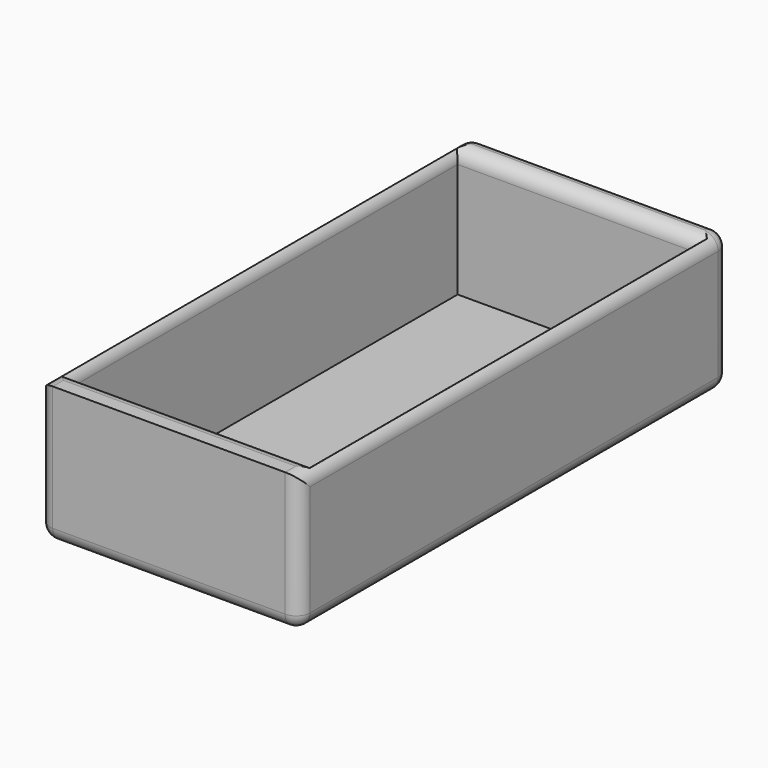
from build123d import *

# Parameters (mm, degrees)
F0_W          = 95.25
F0_H          = 196.85
F1_DEPTH      = 50.8
F2_W          = 87.2193016112
F2_H          = 177.3245334625
F3_DEPTH      = 46.99
F4_T1_DEPTH   = 204.47
F4_T3_DEPTH   = 85.09
F4_T5_DEPTH   = 40.64
F4_T7_DEPTH   = 186.69
F4_T9_DEPTH   = 58.42
F4_T11_DEPTH  = 87.2193016112
F4_T13_DEPTH  = 177.3245334625
F4_S17_W      = 5.1816
F4_S17_H      = 5.1816
F4_T18_DEPTH  = 5.1816
F4_S23_W      = 5.1816
F4_S23_H      = 5.1816
F4_T24_DEPTH  = 5.1816
F4_S29_W      = 5.1816
F4_S29_H      = 5.1816
F4_T30_DEPTH  = 5.1816
F4_S35_W      = 5.1816
F4_S35_H      = 5.1816
F4_T36_DEPTH  = 5.1816
F4_S41_W      = 5.1816
F4_S41_H      = 5.1816
F4_T42_DEPTH  = 5.1816
F4_S47_W      = 5.1816
F4_S47_H      = 5.1816
F4_T48_DEPTH  = 5.1816
F4_T55_DEPTH  = 99.9193016112
F4_T60_DEPTH  = 190.0245334625
F4_T69_DEPTH  = 99.9193016112
F4_T74_DEPTH  = 190.0245334625
F4_T83_DEPTH  = 190.0245334625
F4_T89_DEPTH  = 99.9193016112
F4_T97_DEPTH  = 99.9193016112
F4_T102_DEPTH = 190.0245334625


# Not quite as in the source:
# - a fillet or chamfer that OpenCascade refuses, or shapes differently, is made with other operations: its cross-section is extruded or revolved along the edge and cut away or added


with BuildPart() as f1:
    # F0 (on Top) → F1 (new body)
    with BuildSketch(Plane.XY):
        Rectangle(F0_W, F0_H)
    extrude(amount=F1_DEPTH)

    # F2 (on face) → F3 (cut)
    with BuildSketch(Plane.XY.offset(50.8)):
        with Locations((-0.4809889942, 0.1569911838)):
            Rectangle(F2_W, F2_H)
    extrude(amount=-F3_DEPTH, mode=Mode.SUBTRACT)

    # F4: fillet of radius 5.08 on 15 edges, made by hand

    # F4_s2 → F4_t1 (cut)
    with BuildSketch(Plane.XZ.offset(-93.345)):
        with BuildLine():
            ThreePointArc((-47.625, 45.72), (-46.1371024484, 49.3121024484), (-42.545, 50.8))
            Line((-42.545, 50.8), (-47.625, 50.8))
            Line((-47.625, 50.8), (-47.625, 45.72))
        make_face()
        with BuildLine():
            ThreePointArc((47.625, 45.72), (46.1371024484, 49.3121024484), (42.545, 50.8))
            Line((42.545, 50.8), (47.625, 50.8))
            Line((47.625, 50.8), (47.625, 45.72))
        make_face()
    extrude(amount=F4_T1_DEPTH, mode=Mode.SUBTRACT)

    # F4_s4 → F4_t3 (cut)
    with BuildSketch(Plane.YZ.offset(-42.545)):
        with BuildLine():
            ThreePointArc((98.425, 45.72), (96.9371024484, 49.3121024484), (93.345, 50.8))
            Line((93.345, 50.8), (98.425, 50.8))
            Line((98.425, 50.8), (98.425, 45.72))
        make_face()
        with BuildLine():
            ThreePointArc((-93.345, 0), (-96.9371024484, 1.4878975516), (-98.425, 5.08))
            Line((-98.425, 5.08), (-98.425, 0))
            Line((-98.425, 0), (-93.345, 0))
        make_face()
        with BuildLine():
            ThreePointArc((98.425, 5.08), (96.9371024484, 1.4878975516), (93.345, 0))
            Line((93.345, 0), (98.425, 0))
            Line((98.425, 0), (98.425, 5.08))
        make_face()
    extrude(amount=F4_T3_DEPTH, mode=Mode.SUBTRACT)

    # F4_s6 → F4_t5 (cut)
    with BuildSketch(Plane.XY.offset(5.08)):
        with BuildLine():
            ThreePointArc((-42.545, 98.425), (-46.1371024484, 96.9371024484), (-47.625, 93.345))
            Line((-47.625, 93.345), (-47.625, 98.425))
            Line((-47.625, 98.425), (-42.545, 98.425))
        make_face()
        with BuildLine():
            ThreePointArc((42.545, 98.425), (46.1371024484, 96.9371024484), (47.625, 93.345))
            Line((47.625, 93.345), (47.625, 98.425))
            Line((47.625, 98.425), (42.545, 98.425))
        make_face()
    extrude(amount=F4_T5_DEPTH, mode=Mode.SUBTRACT)

    # F4_s8 → F4_t7 (cut)
    with BuildSketch(Plane.XZ.offset(-93.345)):
        with BuildLine():
            ThreePointArc((-47.625, 5.08), (-46.1371024484, 1.4878975516), (-42.545, 0))
            Line((-42.545, 0), (-47.625, 0))
            Line((-47.625, 0), (-47.625, 5.08))
        make_face()
        with BuildLine():
            ThreePointArc((47.625, 5.08), (46.1371024484, 1.4878975516), (42.545, 0))
            Line((42.545, 0), (47.625, 0))
            Line((47.625, 0), (47.625, 5.08))
        make_face()
    extrude(amount=F4_T7_DEPTH, mode=Mode.SUBTRACT)

    # F4_s10 → F4_t9 (cut)
    with BuildSketch(Plane.XY.offset(5.08)):
        with BuildLine():
            ThreePointArc((-47.625, -93.345), (-46.1371024484, -96.9371024484), (-42.545, -98.425))
            Line((-42.545, -98.425), (-47.625, -98.425))
            Line((-47.625, -98.425), (-47.625, -93.345))
        make_face()
        with BuildLine():
            ThreePointArc((47.625, -93.345), (46.1371024484, -96.9371024484), (42.545, -98.425))
            Line((42.545, -98.425), (47.625, -98.425))
            Line((47.625, -98.425), (47.625, -93.345))
        make_face()
    extrude(amount=F4_T9_DEPTH, mode=Mode.SUBTRACT)

    # F4_s12 → F4_t11 (cut)
    with BuildSketch(Plane.YZ.offset(-44.0906397998)):
        with BuildLine():
            ThreePointArc((93.899257915, 50.8), (90.3071554666, 49.3121024484), (88.819257915, 45.72))
            Line((88.819257915, 45.72), (88.819257915, 50.8))
            Line((88.819257915, 50.8), (93.899257915, 50.8))
        make_face()
        with BuildLine():
            ThreePointArc((-93.5852755475, 50.8), (-89.9931730991, 49.3121024484), (-88.5052755475, 45.72))
            Line((-88.5052755475, 45.72), (-88.5052755475, 50.8))
            Line((-88.5052755475, 50.8), (-93.5852755475, 50.8))
        make_face()
    extrude(amount=F4_T11_DEPTH, mode=Mode.SUBTRACT)

    # F4_s14 → F4_t13 (cut)
    with BuildSketch(Plane.XZ.offset(-88.819257915)):
        with BuildLine():
            ThreePointArc((-49.1706397998, 50.8), (-45.5785373514, 49.3121024484), (-44.0906397998, 45.72))
            Line((-44.0906397998, 45.72), (-44.0906397998, 50.8))
            Line((-44.0906397998, 50.8), (-49.1706397998, 50.8))
        make_face()
        with BuildLine():
            ThreePointArc((48.2086618114, 50.8), (44.6165593629, 49.3121024484), (43.1286618114, 45.72))
            Line((43.1286618114, 45.72), (43.1286618114, 50.8))
            Line((43.1286618114, 50.8), (48.2086618114, 50.8))
        make_face()
    extrude(amount=F4_T13_DEPTH, mode=Mode.SUBTRACT)


with BuildPart() as f4_tool16:
    # F4_s17 → F4_t18 (new body)
    with BuildSketch(Plane.XZ.offset(-93.345)):
        with Locations((-45.1358, 48.3108)):
            Rectangle(F4_S17_W, F4_S17_H)
    extrude(amount=-F4_T18_DEPTH)

    # F4_s19 → F4_t20 (revolve, cut)
    with BuildSketch(Plane(origin=(-42.545, 93.345, 45.72), x_dir=(0.7071067812, 0, -0.7071067812), z_dir=(0.7071067812, 0, 0.7071067812))):
        with BuildLine():
            ThreePointArc((0, -5.08), (5.08, 0), (0, 5.08))
            Line((0, 5.08), (0, -5.08))
        make_face()
    revolve(axis=Axis((-42.545, 93.345, 45.72), (0, 1, 0)), mode=Mode.SUBTRACT)


with BuildPart() as f1_1:
    add(f1.part)

    # F4_t15: cut F4_tool16
    add(f4_tool16.part, mode=Mode.SUBTRACT)


with BuildPart() as f4_tool22:
    # F4_s23 → F4_t24 (new body)
    with BuildSketch(Plane.XZ.offset(-93.345)):
        with Locations((45.1358, 48.3108)):
            Rectangle(F4_S23_W, F4_S23_H)
    extrude(amount=-F4_T24_DEPTH)

    # F4_s25 → F4_t26 (revolve, cut)
    with BuildSketch(Plane(origin=(42.545, 93.345, 45.72), x_dir=(-0.7071067812, 0, -0.7071067812), z_dir=(0.7071067812, 0, -0.7071067812))):
        with BuildLine():
            ThreePointArc((0, -5.08), (5.08, 0), (0, 5.08))
            Line((0, 5.08), (0, -5.08))
        make_face()
    revolve(axis=Axis((42.545, 93.345, 45.72), (0, 1, 0)), mode=Mode.SUBTRACT)


with BuildPart() as f1_2:
    add(f1_1.part)

    # F4_t21: cut F4_tool22
    add(f4_tool22.part, mode=Mode.SUBTRACT)


with BuildPart() as f4_tool28:
    # F4_s29 → F4_t30 (new body)
    with BuildSketch(Plane.XZ.offset(-93.345)):
        with Locations((-45.1358, 2.4892)):
            Rectangle(F4_S29_W, F4_S29_H)
    extrude(amount=-F4_T30_DEPTH)

    # F4_s31 → F4_t32 (revolve, cut)
    with BuildSketch(Plane(origin=(-42.545, 93.345, 5.08), x_dir=(0.7071067812, 0, 0.7071067812), z_dir=(-0.7071067812, 0, 0.7071067812))):
        with BuildLine():
            ThreePointArc((0, -5.08), (5.08, 0), (0, 5.08))
            Line((0, 5.08), (0, -5.08))
        make_face()
    revolve(axis=Axis((-42.545, 93.345, 5.08), (0, 1, 0)), mode=Mode.SUBTRACT)


with BuildPart() as f1_3:
    add(f1_2.part)

    # F4_t27: cut F4_tool28
    add(f4_tool28.part, mode=Mode.SUBTRACT)


with BuildPart() as f4_tool34:
    # F4_s35 → F4_t36 (new body)
    with BuildSketch(Plane.YZ.offset(-42.545)):
        with Locations((-95.9358, 2.4892)):
            Rectangle(F4_S35_W, F4_S35_H)
    extrude(amount=-F4_T36_DEPTH)

    # F4_s37 → F4_t38 (revolve, cut)
    with BuildSketch(Plane(origin=(-42.545, -93.345, 5.08), x_dir=(0, 0.7071067812, 0.7071067812), z_dir=(0, -0.7071067812, 0.7071067812))):
        with BuildLine():
            ThreePointArc((0, -5.08), (5.08, 0), (0, 5.08))
            Line((0, 5.08), (0, -5.08))
        make_face()
    revolve(axis=Axis((-42.545, -93.345, 5.08), (-1, 0, 0)), mode=Mode.SUBTRACT)


with BuildPart() as f1_4:
    add(f1_3.part)

    # F4_t33: cut F4_tool34
    add(f4_tool34.part, mode=Mode.SUBTRACT)


with BuildPart() as f4_tool40:
    # F4_s41 → F4_t42 (new body)
    with BuildSketch(Plane.YZ.offset(42.545)):
        with Locations((-95.9358, 2.4892)):
            Rectangle(F4_S41_W, F4_S41_H)
    extrude(amount=F4_T42_DEPTH)

    # F4_s43 → F4_t44 (revolve, cut)
    with BuildSketch(Plane(origin=(42.545, -93.345, 5.08), x_dir=(0, 0.7071067812, 0.7071067812), z_dir=(0, 0.7071067812, -0.7071067812))):
        with BuildLine():
            ThreePointArc((0, -5.08), (5.08, 0), (0, 5.08))
            Line((0, 5.08), (0, -5.08))
        make_face()
    revolve(axis=Axis((42.545, -93.345, 5.08), (1, 0, 0)), mode=Mode.SUBTRACT)


with BuildPart() as f1_5:
    add(f1_4.part)

    # F4_t39: cut F4_tool40
    add(f4_tool40.part, mode=Mode.SUBTRACT)


with BuildPart() as f4_tool46:
    # F4_s47 → F4_t48 (new body)
    with BuildSketch(Plane.XZ.offset(-93.345)):
        with Locations((45.1358, 2.4892)):
            Rectangle(F4_S47_W, F4_S47_H)
    extrude(amount=-F4_T48_DEPTH)

    # F4_s49 → F4_t50 (revolve, cut)
    with BuildSketch(Plane(origin=(42.545, 93.345, 5.08), x_dir=(-0.7071067812, 0, 0.7071067812), z_dir=(-0.7071067812, 0, -0.7071067812))):
        with BuildLine():
            ThreePointArc((0, -5.08), (5.08, 0), (0, 5.08))
            Line((0, 5.08), (0, -5.08))
        make_face()
    revolve(axis=Axis((42.545, 93.345, 5.08), (0, 1, 0)), mode=Mode.SUBTRACT)


with BuildPart() as f1_6:
    add(f1_5.part)

    # F4_t45: cut F4_tool46
    add(f4_tool46.part, mode=Mode.SUBTRACT)


with BuildPart() as f4_tool53:
    # F4_s54 → F4_t55 (new body)
    with BuildSketch(Plane.YZ.offset(55.8286618114)):
        with BuildLine():
            ThreePointArc((93.899257915, 50.8), (90.3071554666, 49.3121024484), (88.819257915, 45.72))
            Line((88.819257915, 45.72), (88.819257915, 50.8))
            Line((88.819257915, 50.8), (93.899257915, 50.8))
        make_face()
    extrude(amount=-F4_T55_DEPTH)

    split(bisect_by=Plane.YZ.offset(47.625), keep=Keep.BOTTOM)

    split(bisect_by=Plane.YZ.offset(43.1286618114), keep=Keep.TOP)


with BuildPart() as f4_tool58:
    # F4_s59 → F4_t60 (new body)
    with BuildSketch(Plane.XZ.offset(88.5052755475)):
        with BuildLine():
            ThreePointArc((48.2086618114, 50.8), (44.6165593629, 49.3121024484), (43.1286618114, 45.72))
            Line((43.1286618114, 45.72), (43.1286618114, 50.8))
            Line((43.1286618114, 50.8), (48.2086618114, 50.8))
        make_face()
    extrude(amount=-F4_T60_DEPTH)

    split(bisect_by=Plane.XZ.offset(-98.425), keep=Keep.TOP)

    split(bisect_by=Plane.YZ.offset(47.625), keep=Keep.BOTTOM)

    split(bisect_by=Plane.XZ.offset(-88.819257915), keep=Keep.BOTTOM)


with BuildPart() as f4_tool53_1:
    add(f4_tool53.part)

    # F4_t64: intersect F4_tool58
    add(f4_tool58.part, mode=Mode.INTERSECT)


with BuildPart() as f1_7:
    add(f1_6.part)

    # F4_t51: cut F4_tool53
    add(f4_tool53_1.part, mode=Mode.SUBTRACT)


with BuildPart() as f4_tool67:
    # F4_s68 → F4_t69 (new body)
    with BuildSketch(Plane.YZ.offset(43.1286618114)):
        with BuildLine():
            ThreePointArc((93.899257915, 50.8), (90.3071554666, 49.3121024484), (88.819257915, 45.72))
            Line((88.819257915, 45.72), (88.819257915, 50.8))
            Line((88.819257915, 50.8), (93.899257915, 50.8))
        make_face()
    extrude(amount=-F4_T69_DEPTH)

    split(bisect_by=Plane.YZ.offset(-47.625), keep=Keep.TOP)

    split(bisect_by=Plane.YZ.offset(-44.0906397998), keep=Keep.BOTTOM)


with BuildPart() as f4_tool72:
    # F4_s73 → F4_t74 (new body)
    with BuildSketch(Plane.XZ.offset(-101.519257915)):
        with BuildLine():
            ThreePointArc((-49.1706397998, 50.8), (-45.5785373514, 49.3121024484), (-44.0906397998, 45.72))
            Line((-44.0906397998, 45.72), (-44.0906397998, 50.8))
            Line((-44.0906397998, 50.8), (-49.1706397998, 50.8))
        make_face()
    extrude(amount=F4_T74_DEPTH)

    split(bisect_by=Plane.XZ.offset(-98.425), keep=Keep.TOP)

    split(bisect_by=Plane.YZ.offset(-47.625), keep=Keep.TOP)

    split(bisect_by=Plane.XZ.offset(-88.819257915), keep=Keep.BOTTOM)


with BuildPart() as f4_tool67_1:
    add(f4_tool67.part)

    # F4_t78: intersect F4_tool72
    add(f4_tool72.part, mode=Mode.INTERSECT)


with BuildPart() as f1_8:
    add(f1_7.part)

    # F4_t65: cut F4_tool67
    add(f4_tool67_1.part, mode=Mode.SUBTRACT)


with BuildPart() as f4_tool81:
    # F4_s82 → F4_t83 (new body)
    with BuildSketch(Plane.XZ.offset(-88.819257915)):
        with BuildLine():
            ThreePointArc((-49.1706397998, 50.8), (-45.5785373514, 49.3121024484), (-44.0906397998, 45.72))
            Line((-44.0906397998, 45.72), (-44.0906397998, 50.8))
            Line((-44.0906397998, 50.8), (-49.1706397998, 50.8))
        make_face()
    extrude(amount=F4_T83_DEPTH)

    split(bisect_by=Plane.YZ.offset(-47.625), keep=Keep.TOP)

    split(bisect_by=Plane.XZ.offset(98.425), keep=Keep.BOTTOM)

    split(bisect_by=Plane.XZ.offset(88.5052755475), keep=Keep.TOP)


with BuildPart() as f4_tool87:
    # F4_s88 → F4_t89 (new body)
    with BuildSketch(Plane.YZ.offset(-56.7906397998)):
        with BuildLine():
            ThreePointArc((-93.5852755475, 50.8), (-89.9931730991, 49.3121024484), (-88.5052755475, 45.72))
            Line((-88.5052755475, 45.72), (-88.5052755475, 50.8))
            Line((-88.5052755475, 50.8), (-93.5852755475, 50.8))
        make_face()
    extrude(amount=F4_T89_DEPTH)

    split(bisect_by=Plane.YZ.offset(-47.625), keep=Keep.TOP)

    split(bisect_by=Plane.YZ.offset(-44.0906397998), keep=Keep.BOTTOM)


with BuildPart() as f4_tool81_1:
    add(f4_tool81.part)

    # F4_t92: intersect F4_tool87
    add(f4_tool87.part, mode=Mode.INTERSECT)


with BuildPart() as f1_9:
    add(f1_8.part)

    # F4_t79: cut F4_tool81
    add(f4_tool81_1.part, mode=Mode.SUBTRACT)


with BuildPart() as f4_tool95:
    # F4_s96 → F4_t97 (new body)
    with BuildSketch(Plane.YZ.offset(-44.0906397998)):
        with BuildLine():
            ThreePointArc((-93.5852755475, 50.8), (-89.9931730991, 49.3121024484), (-88.5052755475, 45.72))
            Line((-88.5052755475, 45.72), (-88.5052755475, 50.8))
            Line((-88.5052755475, 50.8), (-93.5852755475, 50.8))
        make_face()
    extrude(amount=F4_T97_DEPTH)

    split(bisect_by=Plane.YZ.offset(47.625), keep=Keep.BOTTOM)

    split(bisect_by=Plane.YZ.offset(43.1286618114), keep=Keep.TOP)


with BuildPart() as f4_tool100:
    # F4_s101 → F4_t102 (new body)
    with BuildSketch(Plane.XZ.offset(101.2052755475)):
        with BuildLine():
            ThreePointArc((48.2086618114, 50.8), (44.6165593629, 49.3121024484), (43.1286618114, 45.72))
            Line((43.1286618114, 45.72), (43.1286618114, 50.8))
            Line((43.1286618114, 50.8), (48.2086618114, 50.8))
        make_face()
    extrude(amount=-F4_T102_DEPTH)

    split(bisect_by=Plane.YZ.offset(47.625), keep=Keep.BOTTOM)

    split(bisect_by=Plane.XZ.offset(98.425), keep=Keep.BOTTOM)

    split(bisect_by=Plane.XZ.offset(88.5052755475), keep=Keep.TOP)


with BuildPart() as f4_tool95_1:
    add(f4_tool95.part)

    # F4_t106: intersect F4_tool100
    add(f4_tool100.part, mode=Mode.INTERSECT)


with BuildPart() as f1_10:
    add(f1_9.part)

    # F4_t93: cut F4_tool95
    add(f4_tool95_1.part, mode=Mode.SUBTRACT)


solid = f1_10.part
